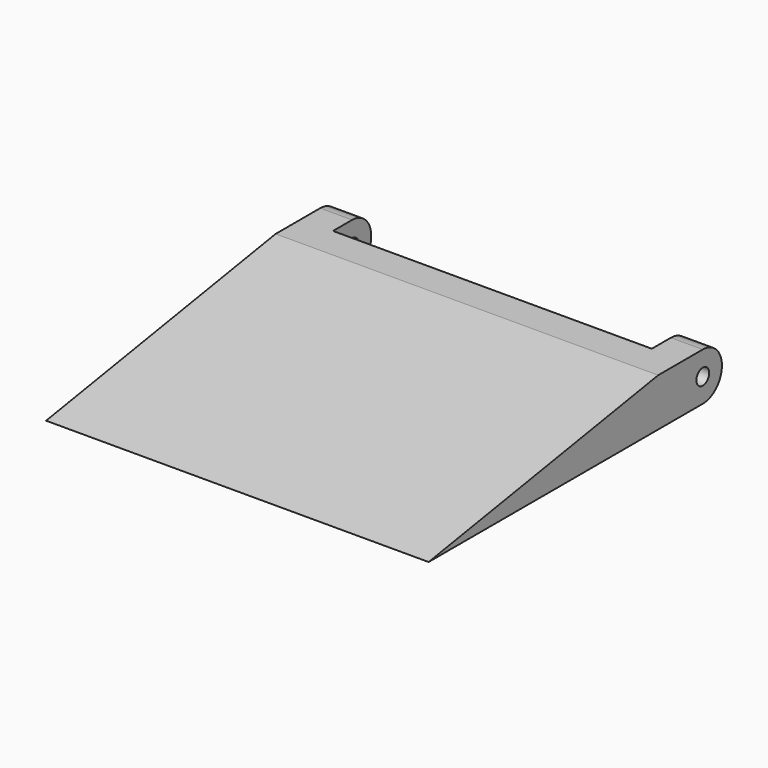
from build123d import *

# Parameters (mm, degrees)
F0_W     = 120
F0_H     = 115
F1_DEPTH = 15
F2_W     = 100
F2_H     = 15
F3_DEPTH = 15.001
F4_R     = 2.5
F5_DEPTH = 120.001
F6_SIZE2 = 14.99999
F6_SIZE  = 89.99999
F7_R     = 7.49999


# Not quite as in the source:
# - a fillet or chamfer is up to 0.001 mm smaller than in the source, because OpenCascade refuses the exact size


with BuildPart() as f1:
    # F0 (on Top) → F1 (new body)
    with BuildSketch(Plane.XY):
        Rectangle(F0_W, F0_H)
    extrude(amount=F1_DEPTH)

    # F2 (on face) → F3 (cut, through all)
    with BuildSketch(Plane.XY.offset(15)):
        with Locations((0, 50)):
            Rectangle(F2_W, F2_H)
    extrude(amount=-F3_DEPTH, mode=Mode.SUBTRACT)

    # F4 (on face) → F5 (cut, through all)
    with BuildSketch(Plane.YZ.offset(60)):
        with Locations((50, 7.5)):
            Circle(F4_R)
    extrude(amount=-F5_DEPTH, mode=Mode.SUBTRACT)

    # F6 (size 90 and 15 in the source; OpenCascade refuses exactly that, so slightly less here)
    f6_edges = [f1.edges().sort_by_distance(p)[0] for p in [
        (0, -57.5, 15),
    ]]
    f6_side = f1.faces().sort_by_distance((0, -6.097561, 15))[0]
    chamfer(f6_edges, length=F6_SIZE, length2=F6_SIZE2, reference=f6_side)

    # F7 (radius 7.5 in the source; OpenCascade refuses exactly that, so slightly less here)
    f7_edges = [f1.edges().sort_by_distance(p)[0] for p in [
        (55, 57.5, 15),
        (55, 57.5, 0),
        (-55, 57.5, 0),
        (-55, 57.5, 15),
    ]]
    fillet(f7_edges, radius=F7_R)


solid = f1.part
